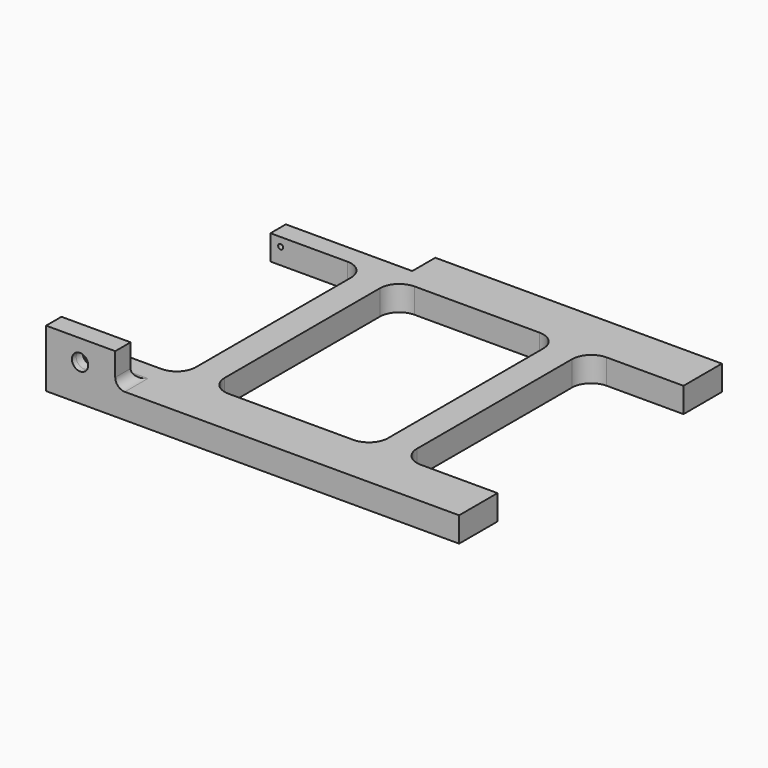
from build123d import *

# Parameters (mm, degrees)
F0_W      = 36
F0_H      = 10
F1_DEPTH  = 13
F3_R      = 2
F4_DEPTH  = 10
F4_TAPER  = 4
F5_DEPTH  = 30
F6_R      = 5
F8_R      = 4.25
F9_DEPTH  = 12.5
F8_R_2    = 4.5
F10_DEPTH = 2.25


# Not quite as in the source:
# - a feature names something its author has since deleted; it is built from what else it names


with BuildPart() as f1:
    # F0 (on Top) → F1 (new body)
    with BuildSketch(Plane.XY):
        with BuildLine():
            Line((-41.7, 85.5), (-41.7, 70.5))
            Line((-41.7, 70.5), (-107.5, 70.5))
            Line((-107.5, 70.5), (-107.5, 60.5))
            Line((-107.5, 60.5), (-67.5, 60.5))
            ThreePointArc((-67.5, 60.5), (-60.4289321881, 57.5710678119), (-57.5, 50.5))
            Line((-57.5, 50.5), (-57.5, -50.5))
            ThreePointArc((-57.5, -50.5), (-60.4289321881, -57.5710678119), (-67.5, -60.5))
            Line((-67.5, -60.5), (-107.5, -60.5))
            Line((-107.5, -60.5), (-107.5, -70.5))
            Line((-107.5, -70.5), (-107.5, -75.5))
            Line((-107.5, -75.5), (-71.5, -75.5))
            Line((-71.5, -75.5), (-71.5, -85.5))
            Line((-71.5, -85.5), (41.7, -85.5))
            Line((41.7, -85.5), (107.5, -85.5))
            Line((107.5, -85.5), (107.5, -70.5))
            Line((107.5, -70.5), (107.5, -60.5))
            Line((107.5, -60.5), (67.5, -60.5))
            ThreePointArc((67.5, -60.5), (60.4289321881, -57.5710678119), (57.5, -50.5))
            Line((57.5, -50.5), (57.5, 50.5))
            ThreePointArc((57.5, 50.5), (60.4289321881, 57.5710678119), (67.5, 60.5))
            Line((67.5, 60.5), (107.5, 60.5))
            Line((107.5, 60.5), (107.5, 70.5))
            Line((107.5, 70.5), (107.5, 85.5))
            Line((107.5, 85.5), (-41.7, 85.5))
        make_face()
        with BuildLine():
            Line((-32.5, 60.5), (32.5, 60.5))
            ThreePointArc((32.5, 60.5), (39.5710678119, 57.5710678119), (42.5, 50.5))
            Line((42.5, 50.5), (42.5, -50.5))
            ThreePointArc((42.5, -50.5), (39.5710678119, -57.5710678119), (32.5, -60.5))
            Line((32.5, -60.5), (-32.5, -60.5))
            ThreePointArc((-32.5, -60.5), (-39.5710678119, -57.5710678119), (-42.5, -50.5))
            Line((-42.5, -50.5), (-42.5, 50.5))
            ThreePointArc((-42.5, 50.5), (-39.5710678119, 57.5710678119), (-32.5, 60.5))
        make_face(mode=Mode.SUBTRACT)
        with Locations((-89.5, -80.5)):
            Rectangle(F0_W, F0_H)
    extrude(amount=F1_DEPTH)

    # F3 (on offset) → F4 (cut)
    with BuildSketch(Plane(origin=(0, 70.5, 0), x_dir=(-1, 0, 0), z_dir=(0, 1, 0))):
        with Locations((47.2, 6)):
            Circle(F3_R)
        with Locations((102.2, 8.5)):
            Circle(F3_R)
    extrude(amount=-F4_DEPTH, taper=F4_TAPER, mode=Mode.SUBTRACT)

    # F0 (on Top) → F5 (join)
    with BuildSketch(Plane.XY):
        with Locations((-89.5, -80.5)):
            Rectangle(F0_W, F0_H)
    extrude(amount=F5_DEPTH)

    # F6
    f6_edges = [f1.edges().sort_by_distance(p)[0] for p in [
        (-89.5, -75.5, 13),
        (-71.5, -80.5, 13),
    ]]
    fillet(f6_edges, radius=F6_R)

    # F8 (on offset) → F9 (cut, symmetric)
    with BuildSketch(Plane.XZ.offset(80.5)):
        with Locations((-89.8, 19)):
            Circle(F8_R)
    extrude(amount=F9_DEPTH, both=True, mode=Mode.SUBTRACT)

    # F8 (on offset) → F10 (cut, symmetric)
    with BuildSketch(Plane.XZ.offset(80.5)):
        with Locations((-89.8, 19)):
            Circle(F8_R_2)
        with Locations((-89.8, 19)):
            Circle(F8_R, mode=Mode.SUBTRACT)
    extrude(amount=F10_DEPTH, both=True, mode=Mode.SUBTRACT)


solid = f1.part
